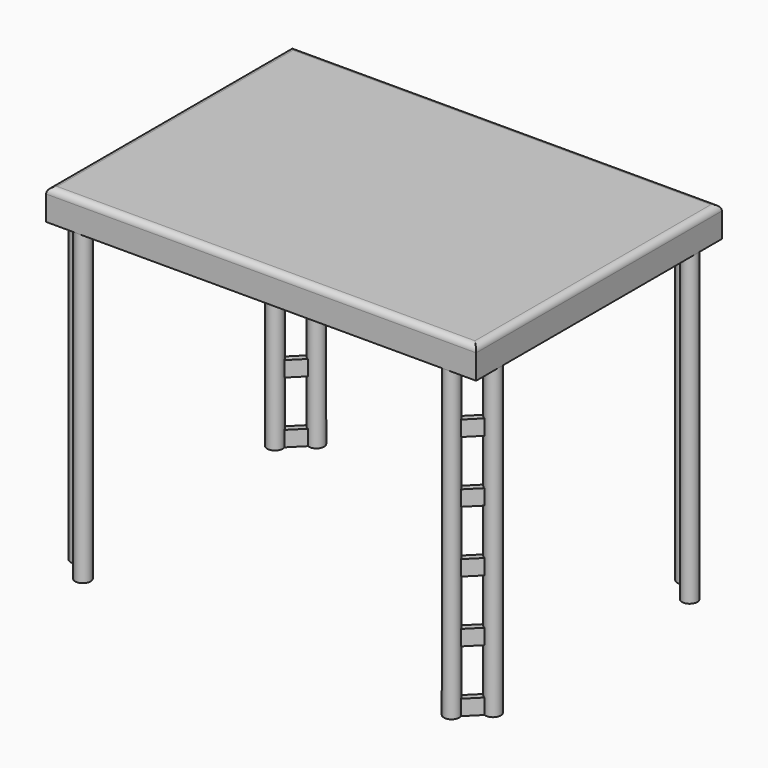
from build123d import *

# Parameters (mm, degrees)
F0_W         = 177.8
F0_H         = 127
F1_DEPTH     = 12.7
F2_R         = 3.175
F3_DEPTH     = 127
F6_W         = 13.4703841816
F6_H         = 6.35
F7_DEPTH     = 1.27
F8_R         = 2.54
F9_T1_DEPTH  = 10.16
F9_T3_DEPTH  = 7.62
F9_T5_DEPTH  = 10.1599999705
F9_S9_W      = 2.54
F9_S9_H      = 2.54
F9_T10_DEPTH = 2.54
F9_S15_W     = 2.54
F9_S15_H     = 2.54
F9_T16_DEPTH = 2.54
F9_T22_DEPTH = 171.4500000295
F9_S23_R     = 3.175
F9_T24_DEPTH = 87
F9_T28_DEPTH = 120.65
F9_S29_R     = 3.175
F9_T30_DEPTH = 62


# Not quite as in the source:
# - a fillet or chamfer that OpenCascade refuses, or shapes differently, is made with other operations: its cross-section is extruded or revolved along the edge and cut away or added


with BuildPart() as f1:
    # F0 (on Top) → F1 (new body)
    with BuildSketch(Plane.XY):
        Rectangle(F0_W, F0_H)
    extrude(amount=F1_DEPTH)

    # F2 (on Top) → F3 (join)
    with BuildSketch(Plane.XY):
        with Locations((76.2, -60.325)):
            Circle(F2_R)
        with Locations((85.725, -50.8)):
            Circle(F2_R)
    extrude(amount=-F3_DEPTH)

    # F6 (on face) → F7 (join, symmetric)
    with BuildSketch(Plane(origin=(68.2625, -68.2625, 0), x_dir=(0.7071067812, 0.7071067812, 0), z_dir=(0.7071067812, -0.7071067812, 0))):
        with Locations((17.9605122421, -22.225)):
            Rectangle(F6_W, F6_H)
        with Locations((17.9605122421, -47.625)):
            Rectangle(F6_W, F6_H)
        Polygon((11.2253201513, -76.2), (24.6957043329, -76.2), (24.6957043329, -69.85), (11.2336926315, -69.85), (11.2253201513, -69.85), align=None)
        with Locations((17.9605122421, -98.425)):
            Rectangle(F6_W, F6_H)
        with Locations((17.9605122421, -123.825)):
            Rectangle(F6_W, F6_H)
    extrude(amount=F7_DEPTH, both=True)

    # F8
    f8_edges = [f1.edges().sort_by_distance(p)[0] for p in [
        (0, -63.5, 12.7),
        (88.9, 0, 12.7),
        (0, 63.5, 12.7),
        (-88.9, 0, 12.7),
    ]]
    fillet(f8_edges, radius=F8_R)

    # F9: fillet of radius 2.54 on 3 edges, made by hand

    # F9_s2 → F9_t1 (cut)
    with BuildSketch(Plane.XZ.offset(50.8)):
        with BuildLine():
            ThreePointArc((86.36, 0), (88.1560512242, 0.7439487758), (88.9, 2.54))
            Line((88.9, 2.54), (88.9, 0))
            Line((88.9, 0), (86.36, 0))
        make_face()
    extrude(amount=F9_T1_DEPTH, mode=Mode.SUBTRACT)

    # F9_s4 → F9_t3 (cut)
    with BuildSketch(Plane.XY.offset(2.54)):
        with BuildLine():
            ThreePointArc((86.36, -63.5), (88.1560512242, -62.7560512242), (88.9, -60.96))
            Line((88.9, -60.96), (88.9, -63.5))
            Line((88.9, -63.5), (86.36, -63.5))
        make_face()
    extrude(amount=F9_T3_DEPTH, mode=Mode.SUBTRACT)

    # F9_s6 → F9_t5 (cut)
    with BuildSketch(Plane.YZ.offset(76.2000000295)):
        with BuildLine():
            ThreePointArc((-63.5, 2.54), (-62.7560512242, 0.7439487758), (-60.96, 0))
            Line((-60.96, 0), (-63.5, 0))
            Line((-63.5, 0), (-63.5, 2.54))
        make_face()
    extrude(amount=F9_T5_DEPTH, mode=Mode.SUBTRACT)


with BuildPart() as f9_tool8:
    # F9_s9 → F9_t10 (new body)
    with BuildSketch(Plane.XZ.offset(60.96)):
        with Locations((87.63, 11.43)):
            Rectangle(F9_S9_W, F9_S9_H)
    extrude(amount=F9_T10_DEPTH)

    # F9_s11 → F9_t12 (revolve, cut)
    with BuildSketch(Plane(origin=(86.36, -60.96, 10.16), x_dir=(-0.7071067812, 0, -0.7071067812), z_dir=(-0.7071067812, 0, 0.7071067812))):
        with BuildLine():
            ThreePointArc((0, -2.54), (2.54, 0), (0, 2.54))
            Line((0, 2.54), (0, -2.54))
        make_face()
    revolve(axis=Axis((86.36, -60.96, 10.16), (0, -1, 0)), mode=Mode.SUBTRACT)


with BuildPart() as f1_1:
    add(f1.part)

    # F9_t7: cut F9_tool8
    add(f9_tool8.part, mode=Mode.SUBTRACT)


with BuildPart() as f9_tool14:
    # F9_s15 → F9_t16 (new body)
    with BuildSketch(Plane.XZ.offset(60.96)):
        with Locations((87.63, 1.27)):
            Rectangle(F9_S15_W, F9_S15_H)
    extrude(amount=F9_T16_DEPTH)

    # F9_s17 → F9_t18 (revolve, cut)
    with BuildSketch(Plane(origin=(86.36, -60.96, 2.54), x_dir=(-0.7071067812, 0, 0.7071067812), z_dir=(0.7071067812, 0, 0.7071067812))):
        with BuildLine():
            ThreePointArc((0, -2.54), (2.54, 0), (0, 2.54))
            Line((0, 2.54), (0, -2.54))
        make_face()
    revolve(axis=Axis((86.36, -60.96, 2.54), (0, -1, 0)), mode=Mode.SUBTRACT)


with BuildPart() as f1_2:
    add(f1_1.part)

    # F9_t13: cut F9_tool14
    add(f9_tool14.part, mode=Mode.SUBTRACT)


with BuildPart() as f9_tool20:
    # F9_s21 → F9_t22 (new body)
    with BuildSketch(Plane.YZ.offset(-95.25)):
        with BuildLine():
            ThreePointArc((-63.5, 2.54), (-62.7560512242, 0.7439487758), (-60.96, 0))
            Line((-60.96, 0), (-63.5, 0))
            Line((-63.5, 0), (-63.5, 2.54))
        make_face()
    extrude(amount=F9_T22_DEPTH)

    # F9_s23 → F9_t24 (cut, symmetric)
    with BuildSketch(Plane.XY.offset(1.3)):
        with Locations((76.2, -60.325)):
            Circle(F9_S23_R)
    extrude(amount=F9_T24_DEPTH, both=True, mode=Mode.SUBTRACT)


with BuildPart() as f1_3:
    add(f1_2.part)

    # F9_t19: cut F9_tool20
    add(f9_tool20.part, mode=Mode.SUBTRACT)


with BuildPart() as f9_tool26:
    # F9_s27 → F9_t28 (new body)
    with BuildSketch(Plane.XZ.offset(50.8)):
        with BuildLine():
            ThreePointArc((86.36, 0), (88.1560512242, 0.7439487758), (88.9, 2.54))
            Line((88.9, 2.54), (88.9, 0))
            Line((88.9, 0), (86.36, 0))
        make_face()
    extrude(amount=-F9_T28_DEPTH)

    # F9_s29 → F9_t30 (cut, symmetric)
    with BuildSketch(Plane.XY.offset(1.3)):
        with Locations((85.725, -50.8)):
            Circle(F9_S29_R)
    extrude(amount=F9_T30_DEPTH, both=True, mode=Mode.SUBTRACT)


with BuildPart() as f1_4:
    add(f1_3.part)

    # F9_t25: cut F9_tool26
    add(f9_tool26.part, mode=Mode.SUBTRACT)

    # F10: F1 across plane


with BuildPart() as f1_5:
    add(f1_4.part)
    add(f1_4.part.mirror(Plane.YZ))

    # F11: F1 across plane


with BuildPart() as f1_6:
    add(f1_5.part)
    add(f1_5.part.mirror(Plane.XZ))


solid = f1_6.part
